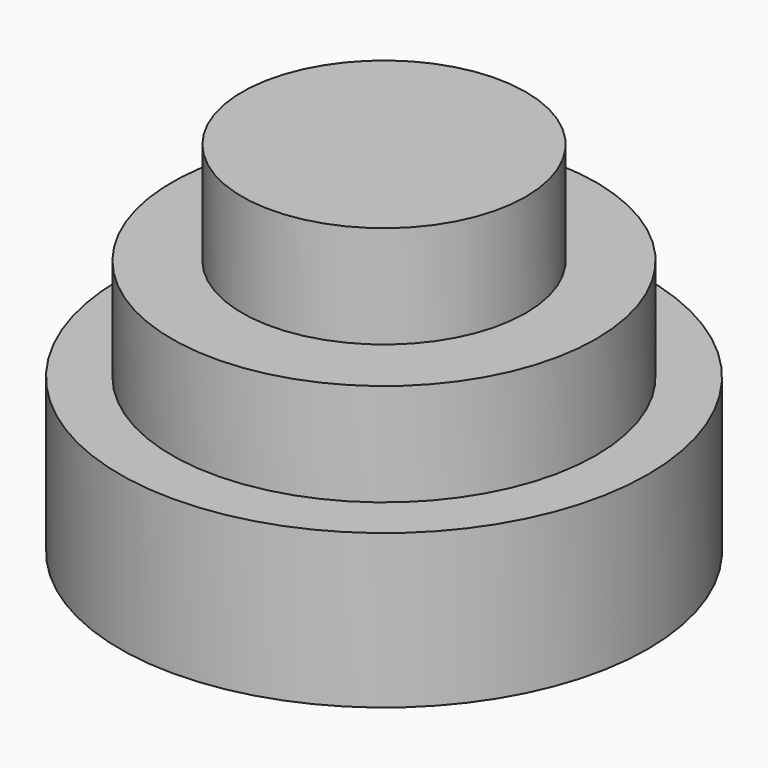
from build123d import *

# Parameters (mm, degrees)
F0_R     = 65.4726096666
F1_DEPTH = 38.1
F2_R     = 52.6067732991
F3_DEPTH = 25.4
F4_R     = 35.1837218131
F5_DEPTH = 25.4


# Not quite as in the source:
# - the program builds the solid bodies; features that only make, move or delete a surface that nothing else refers to are left out


with BuildPart() as f1:
    # F0 (on Top) → F1 (new body)
    with BuildSketch(Plane.XY):
        Circle(F0_R)
    extrude(amount=F1_DEPTH)

    # F2 (on face) → F3 (join)
    with BuildSketch(Plane.XY.offset(38.1)):
        Circle(F2_R)
    extrude(amount=F3_DEPTH)

    # F4 (on face) → F5 (join)
    with BuildSketch(Plane.XY.offset(63.5)):
        Circle(F4_R)
    extrude(amount=F5_DEPTH)


solid = f1.part
